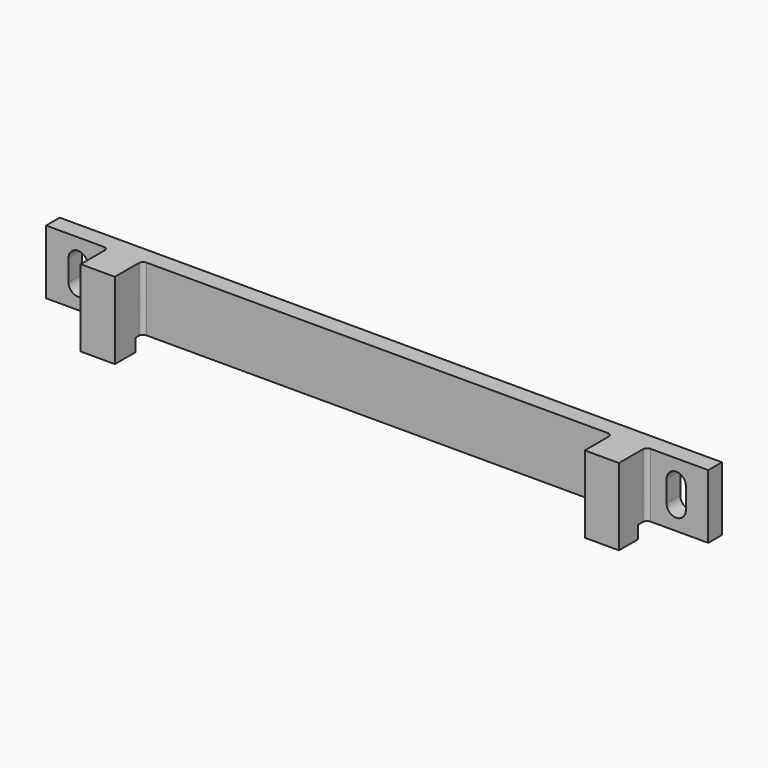
from build123d import *

# Parameters (mm, degrees)
F0_W     = 155
F0_H     = 15
F1_DEPTH = 4
F2_W     = 8
F2_H     = 15
F3_DEPTH = 8
F4_W     = 8
F4_H     = 6
F4_H_2   = 5.5
F5_DEPTH = 3
F6_R     = 1


# Not quite as in the source:
# - a feature names something its author has since deleted; it is built from what else it names


with BuildPart() as f1:
    # F0 (on Front) → F1 (new body)
    with BuildSketch(Plane.XZ):
        Rectangle(F0_W, F0_H)
        with BuildLine():
            Line((-72.25, -2.5), (-72.25, 2.5))
            ThreePointArc((-72.25, 2.5), (-70, 4.75), (-67.75, 2.5))
            Line((-67.75, 2.5), (-67.75, -2.5))
            ThreePointArc((-67.75, -2.5), (-70, -4.75), (-72.25, -2.5))
        make_face(mode=Mode.SUBTRACT)
        with BuildLine():
            ThreePointArc((67.75, 2.5), (70, 4.75), (72.25, 2.5))
            Line((72.25, 2.5), (72.25, -2.5))
            ThreePointArc((72.25, -2.5), (70, -4.75), (67.75, -2.5))
            Line((67.75, -2.5), (67.75, 2.5))
        make_face(mode=Mode.SUBTRACT)
    extrude(amount=F1_DEPTH)

    # F2 (on face) → F3 (join)
    with BuildSketch(Plane.XZ.offset(4)):
        with Locations((-59, 0)):
            Rectangle(F2_W, F2_H)
        with Locations((59, 0)):
            Rectangle(F2_W, F2_H)
    extrude(amount=F3_DEPTH)

    # F4 (on face) → F5 (join)
    with BuildSketch(Plane(origin=(0, 0, -7.5), x_dir=(1, 0, 0), z_dir=(0, 0, -1))):
        with Locations((-59, 9)):
            Rectangle(F4_W, F4_H)
        with Locations((59, 9.25)):
            Rectangle(F4_W, F4_H_2)
    extrude(amount=F5_DEPTH)

    # F6
    f6_edges = [f1.edges().sort_by_distance(p)[0] for p in [
        (55, -4, 0),
        (-55, -4, 0),
        (63, -4, 0),
        (-63, -4, 0),
    ]]
    fillet(f6_edges, radius=F6_R)


solid = f1.part
